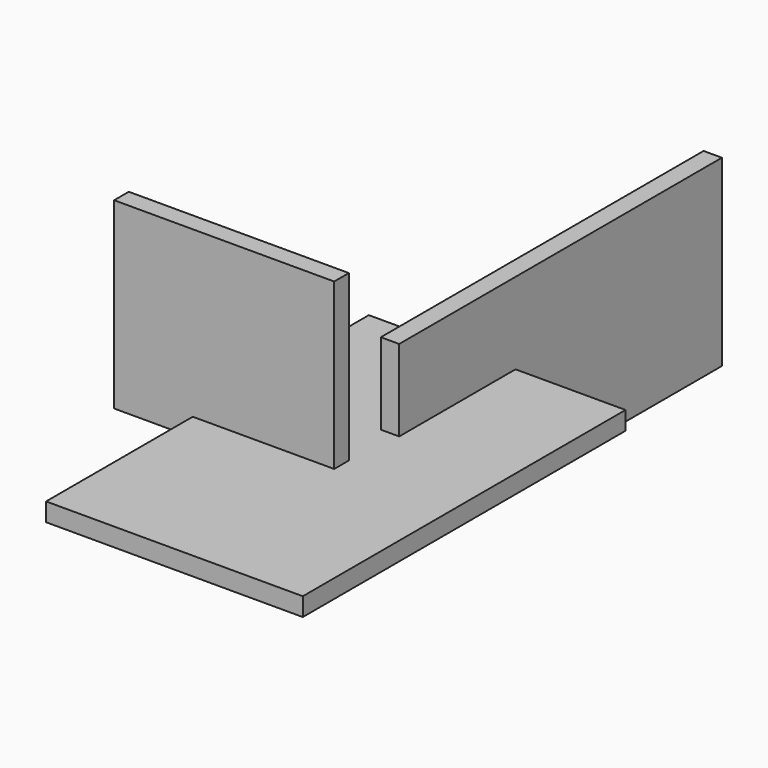
from build123d import *

# Parameters (mm, degrees)
F2_W     = 76.2
F2_H     = 63.5
F3_DEPTH = 6.35
F1_W     = 127
F1_H     = 63.5
F1_W_2   = 6.35
F4_DEPTH = 6.35
F5_DEPTH = 6.35


with BuildPart() as f3:
    # F2 (on Front) → F3 (new body)
    with BuildSketch(Plane.XZ):
        with Locations((-33.5817006469, 31.75)):
            Rectangle(F2_W, F2_H)
    extrude(amount=F3_DEPTH)


with BuildPart() as f4:
    # F1 (on Right) → F4 (new body)
    with BuildSketch(Plane.YZ):
        with Locations((89.3461111993, 2.793211019)):
            Rectangle(F1_W, F1_H)
        with Locations((22.6711111993, 2.793211019)):
            Rectangle(F1_W_2, F1_H)
        with Locations((156.0211111993, 2.793211019)):
            Rectangle(F1_W_2, F1_H)
    extrude(amount=F4_DEPTH)


with BuildPart() as f5:
    # F0 (on Top) → F5 (new body)
    with BuildSketch(Plane.XY):
        Polygon((38.1, 0), (0, 0), (-38.1, 0), (-38.1, -63.5), (0, -63.5), (38.1, -63.5), align=None)
        Polygon((-38.1, 0), (0, 0), (38.1, 0), (38.1, 63.5), (0, 63.5), (-38.1, 63.5), align=None)
        Polygon((-44.45, 0), (-38.1, 0), (-38.1, 63.5), (0, 63.5), (0, 69.85), (-44.45, 69.85), align=None)
        Polygon((-38.1, -63.5), (-38.1, 0), (-44.45, 0), (-44.45, -69.85), (0, -69.85), (0, -63.5), align=None)
        Polygon((44.45, 0), (38.1, 0), (38.1, -63.5), (0, -63.5), (0, -69.85), (44.45, -69.85), align=None)
        Polygon((38.1, 63.5), (38.1, 0), (44.45, 0), (44.45, 69.85), (0, 69.85), (0, 63.5), align=None)
    extrude(amount=F5_DEPTH)


solid = Compound([f3.part, f4.part, f5.part])
